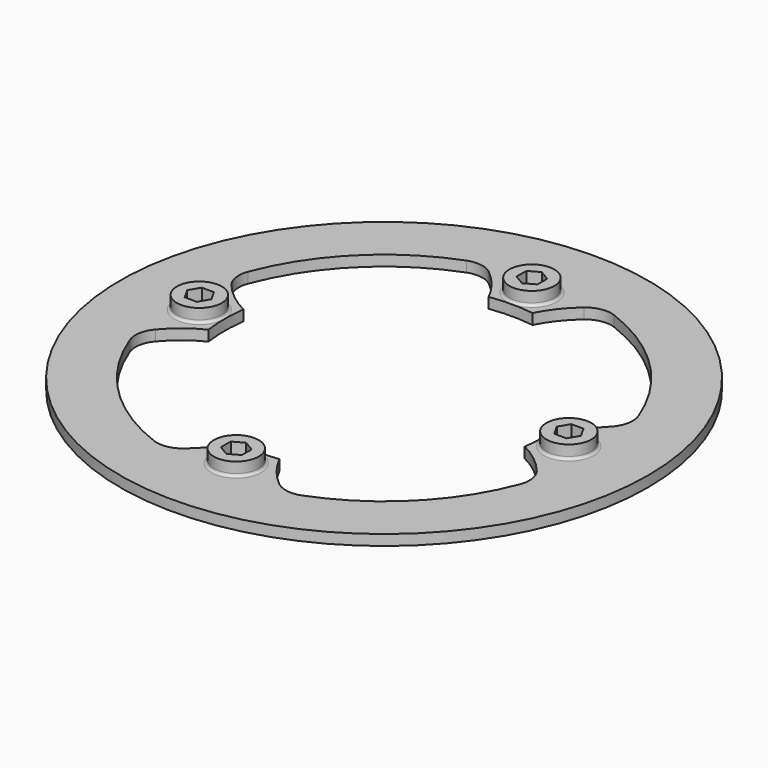
from build123d import *

# Parameters (mm, degrees)
F0_R     = 100
F0_R_2   = 2.5
F1_DEPTH = 4
F2_R     = 8.5
F3_DEPTH = 5
F4_R     = 10
F5_R     = 0.99999


# Not quite as in the source:
# - a fillet or chamfer is up to 0.001 mm smaller than in the source, because OpenCascade refuses the exact size


with BuildPart() as f1:
    # F0 (on Top) → F1 (new body)
    with BuildSketch(Plane.XY):
        Circle(F0_R)
        with BuildLine():
            ThreePointArc((22.8257041117, 75.7052949069), (55.9120042797, 55.9120042797), (75.7052949069, 22.8257041117))
            ThreePointArc((75.7052949069, 22.8257041117), (78.2254331665, 11.536292778), (79.0715147518, 0))
            ThreePointArc((79.0715147518, 0), (78.2254331665, -11.536292778), (75.7052949069, -22.8257041117))
            ThreePointArc((75.7052949069, -22.8257041117), (55.9120042797, -55.9120042797), (22.8257041117, -75.7052949069))
            ThreePointArc((22.8257041117, -75.7052949069), (0, -79.0715147518), (-22.8257041117, -75.7052949069))
            ThreePointArc((-22.8257041117, -75.7052949069), (-55.9120042797, -55.9120042797), (-75.7052949069, -22.8257041117))
            ThreePointArc((-75.7052949069, -22.8257041117), (-79.0715147518, 0), (-75.7052949069, 22.8257041117))
            ThreePointArc((-75.7052949069, 22.8257041117), (-55.9120042797, 55.9120042797), (-22.8257041117, 75.7052949069))
            ThreePointArc((-22.8257041117, 75.7052949069), (0, 79.0715147518), (22.8257041117, 75.7052949069))
        make_face(mode=Mode.SUBTRACT)
        with BuildLine():
            ThreePointArc((-8.3091100857, 59.9266942988), (0, 60.5), (8.3091100857, 59.9266942988))
            ThreePointArc((8.3091100857, 59.9266942988), (14.4468681442, 68.8469104297), (22.8257041117, 75.7052949069))
            ThreePointArc((22.8257041117, 75.7052949069), (0, 79.0715147518), (-22.8257041117, 75.7052949069))
            ThreePointArc((-22.8257041117, 75.7052949069), (-14.4468681442, 68.8469104297), (-8.3091100857, 59.9266942988))
        make_face()
        Polygon((0.2799602618, 74.6188021535), (4.2799602618, 72.3094010768), (4.2799602618, 67.6905989232), (0.2799602618, 65.3811978465), (-3.7200397382, 67.6905989232), (-3.7200397382, 72.3094010768), align=None, mode=Mode.SUBTRACT)
        with BuildLine():
            ThreePointArc((-59.9266942988, -8.3091100857), (-60.5, 0), (-59.9266942988, 8.3091100857))
            ThreePointArc((-59.9266942988, 8.3091100857), (-68.8469104297, 14.4468681442), (-75.7052949069, 22.8257041117))
            ThreePointArc((-75.7052949069, 22.8257041117), (-79.0715147518, 0), (-75.7052949069, -22.8257041117))
            ThreePointArc((-75.7052949069, -22.8257041117), (-68.8469104297, -14.4468681442), (-59.9266942988, -8.3091100857))
        make_face()
        Polygon((-65.3811978465, 0.2799602618), (-67.6905989232, -3.7200397382), (-72.3094010768, -3.7200397382), (-74.6188021535, 0.2799602618), (-72.3094010768, 4.2799602618), (-67.6905989232, 4.2799602618), align=None, mode=Mode.SUBTRACT)
        with BuildLine():
            ThreePointArc((59.9266942988, 8.3091100857), (60.3565033989, 4.1644324296), (60.5, 0))
            ThreePointArc((60.5, 0), (60.3565033989, -4.1644324296), (59.9266942988, -8.3091100857))
            ThreePointArc((59.9266942988, -8.3091100857), (68.8469104297, -14.4468681442), (75.7052949069, -22.8257041117))
            ThreePointArc((75.7052949069, -22.8257041117), (78.2254331665, -11.536292778), (79.0715147518, 0))
            ThreePointArc((79.0715147518, 0), (78.2254331665, 11.536292778), (75.7052949069, 22.8257041117))
            ThreePointArc((75.7052949069, 22.8257041117), (68.8469104297, 14.4468681442), (59.9266942988, 8.3091100857))
        make_face()
        Polygon((74.6188021535, -0.2799602618), (72.3094010768, -4.2799602618), (67.6905989232, -4.2799602618), (65.3811978465, -0.2799602618), (67.6905989232, 3.7200397382), (72.3094010768, 3.7200397382), align=None, mode=Mode.SUBTRACT)
        with BuildLine():
            ThreePointArc((22.8257041117, -75.7052949069), (14.4468681442, -68.8469104297), (8.3091100857, -59.9266942988))
            ThreePointArc((8.3091100857, -59.9266942988), (0, -60.5), (-8.3091100857, -59.9266942988))
            ThreePointArc((-8.3091100857, -59.9266942988), (-14.4468681442, -68.8469104297), (-22.8257041117, -75.7052949069))
            ThreePointArc((-22.8257041117, -75.7052949069), (0, -79.0715147518), (22.8257041117, -75.7052949069))
        make_face()
        Polygon((-0.2799602618, -74.6188021535), (-4.2799602618, -72.3094010768), (-4.2799602618, -67.6905989232), (-0.2799602618, -65.3811978465), (3.7200397382, -67.6905989232), (3.7200397382, -72.3094010768), align=None, mode=Mode.SUBTRACT)
        Polygon((-72.3094010768, -3.7200397382), (-67.6905989232, -3.7200397382), (-65.3811978465, 0.2799602618), (-67.6905989232, 4.2799602618), (-72.3094010768, 4.2799602618), (-74.6188021535, 0.2799602618), align=None)
        with Locations((-70, 0)):
            Circle(F0_R_2, mode=Mode.SUBTRACT)
        Polygon((-4.2799602618, -67.6905989232), (-4.2799602618, -72.3094010768), (-0.2799602618, -74.6188021535), (3.7200397382, -72.3094010768), (3.7200397382, -67.6905989232), (-0.2799602618, -65.3811978465), align=None)
        with Locations((0, -70)):
            Circle(F0_R_2, mode=Mode.SUBTRACT)
        Polygon((67.6905989232, -4.2799602618), (72.3094010768, -4.2799602618), (74.6188021535, -0.2799602618), (72.3094010768, 3.7200397382), (67.6905989232, 3.7200397382), (65.3811978465, -0.2799602618), align=None)
        with Locations((70, 0)):
            Circle(F0_R_2, mode=Mode.SUBTRACT)
        Polygon((4.2799602618, 67.6905989232), (4.2799602618, 72.3094010768), (0.2799602618, 74.6188021535), (-3.7200397382, 72.3094010768), (-3.7200397382, 67.6905989232), (0.2799602618, 65.3811978465), align=None)
        with Locations((0, 70)):
            Circle(F0_R_2, mode=Mode.SUBTRACT)
    extrude(amount=F1_DEPTH)

    # F2 (on face) → F3 (join)
    with BuildSketch(Plane.XY.offset(4)):
        with Locations((-70, 0)):
            Circle(F2_R)
        Polygon((-67.7365000122, -4.0261521504), (-72.3550000478, -3.9733245662), (-74.6185000357, 0.0528275843), (-72.2634999878, 4.0261521504), (-67.6449999522, 3.9733245662), (-65.3814999643, -0.0528275843), align=None, mode=Mode.SUBTRACT)
        with Locations((0, 70)):
            Circle(F2_R)
        Polygon((-4.0261521504, 67.7365000122), (-3.9733245662, 72.3550000478), (0.0528275843, 74.6185000357), (4.0261521504, 72.2634999878), (3.9733245662, 67.6449999522), (-0.0528275843, 65.3814999643), align=None, mode=Mode.SUBTRACT)
        with Locations((70, 0)):
            Circle(F2_R)
        Polygon((67.7365000122, 4.0261521504), (72.3550000478, 3.9733245662), (74.6185000357, -0.0528275843), (72.2634999878, -4.0261521504), (67.6449999522, -3.9733245662), (65.3814999643, 0.0528275843), align=None, mode=Mode.SUBTRACT)
        with Locations((0, -70)):
            Circle(F2_R)
        Polygon((4.0261521504, -67.7365000122), (3.9733245662, -72.3550000478), (-0.0528275843, -74.6185000357), (-4.0261521504, -72.2634999878), (-3.9733245662, -67.6449999522), (0.0528275843, -65.3814999643), align=None, mode=Mode.SUBTRACT)
    extrude(amount=F3_DEPTH)

    # F4
    f4_edges = [f1.edges().sort_by_distance(p)[0] for p in [
        (-75.705295, 22.825704, 2),
        (-75.705295, -22.825704, 2),
        (75.705295, -22.825704, 2),
        (22.825704, -75.705295, 2),
        (-22.825704, -75.705295, 2),
        (75.705295, 22.825704, 2),
        (22.825704, 75.705295, 2),
        (-22.825704, 75.705295, 2),
    ]]
    fillet(f4_edges, radius=F4_R)

    # F5 (radius 1 in the source; OpenCascade refuses exactly that, so slightly less here)
    f5_edges = [f1.edges().sort_by_distance(p)[0] for p in [
        (-8.5, -70, 4),
        (-8.5, 70, 4),
        (-78.5, 0, 4),
        (61.5, 0, 4),
    ]]
    fillet(f5_edges, radius=F5_R)


solid = f1.part
